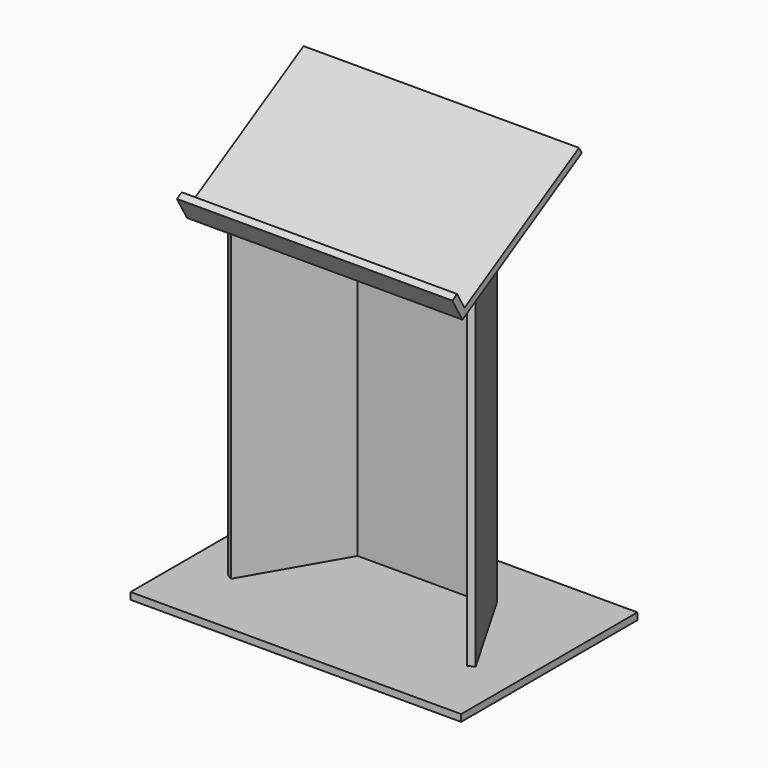
from build123d import *

# Parameters (mm, degrees)
F2_DEPTH = 381
F0_W     = 914.4
F0_H     = 609.6
F3_DEPTH = 19.05
F4_REACH = 1907.1780931


with BuildPart() as f2:
    # F1 (on Right) → F2 (new body, symmetric)
    with BuildSketch(Plane.YZ):
        Polygon((-197.9734073051, 940.2559094878), (-223.3734073051, 984.25), (-239.8711912472, 974.725), (-204.9461912472, 914.2331255457), (207.4984073051, 1152.3581255457), (197.9734073051, 1168.8559094878), align=None)
    extrude(amount=F2_DEPTH, both=True)



with BuildPart() as f3:
    # F0 (on Top) → F3 (new body)
    with BuildSketch(Plane.XY):
        Rectangle(F0_W, F0_H)
        Polygon((-342.9, -111.5645430735), (-190.5, 152.4), (190.5, 152.4), (342.9, -111.5645430735), (326.4022160579, -121.0895430735), (179.5014773719, 133.35), (-179.5014773719, 133.35), (-326.4022160579, -121.0895430735), align=None, mode=Mode.SUBTRACT)
        Polygon((190.5, 152.4), (-190.5, 152.4), (-342.9, -111.5645430735), (-326.4022160579, -121.0895430735), (-179.5014773719, 133.35), (179.5014773719, 133.35), (326.4022160579, -121.0895430735), (342.9, -111.5645430735), align=None)
    extrude(amount=F3_DEPTH)


with BuildPart() as f2_1:
    add(f2.part)

    add(f3.part)  # F4 merges F3
    f4_end = f2_1.faces().sort_by_distance((0, 1.276108029, 1033.2956255457))[0]
    # F0 (on Top) → F4 (join, up to a face of the model that its end follows)
    with BuildSketch(Plane.XY):
        Polygon((190.5, 152.4), (-190.5, 152.4), (-342.9, -111.5645430735), (-326.4022160579, -121.0895430735), (-179.5014773719, 133.35), (179.5014773719, 133.35), (326.4022160579, -121.0895430735), (342.9, -111.5645430735), align=None)
    f4_long = extrude(amount=F4_REACH, mode=Mode.PRIVATE)
    add(split(f4_long, bisect_by=f4_end, keep=Keep.TOP, mode=Mode.PRIVATE))


solid = f2_1.part
